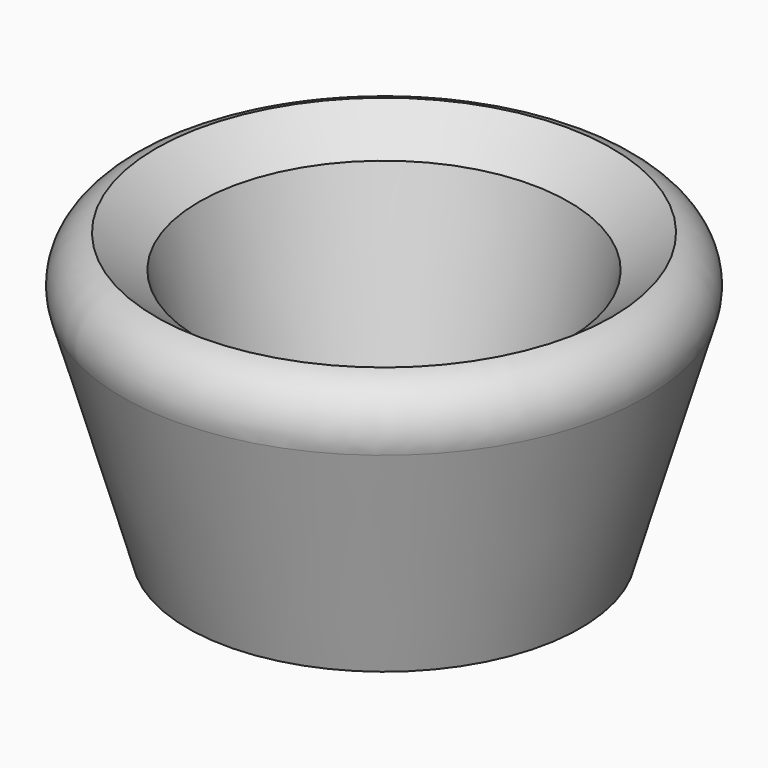
from build123d import *

# Parameters (mm, degrees)
F2_SIZE = 5


# Not quite as in the source:
# - a fillet or chamfer that OpenCascade refuses, or shapes differently, is made with other operations: its cross-section is extruded or revolved along the edge and cut away or added


with BuildPart() as f1:
    # F0 (on Front) → F1 (revolve)
    with BuildSketch(Plane.XZ):
        Polygon((-28.7600811571, 0), (0, 0), (0, 6.0786292888), (-18.5987912118, 6.0786292888), (-28.3971782774, 41.6431464255), (-40.9173406661, 41.6431464255), align=None)
    revolve(axis=Axis((0, 0, 3.0393146444), (0, 0, -1)))

    # F2
    f2_edges = [f1.edges().sort_by_distance(p)[0] for p in [
        (28.397178, 0, 41.643146),
    ]]
    chamfer(f2_edges, length=F2_SIZE)

    # F3: fillet of radius 7 on 1 edges, made by hand

    # F3_s1 → F3_t2 (revolve, cut)
    with BuildSketch(Plane.XZ):
        with BuildLine():
            ThreePointArc((-33.3971782774, 41.6431464255), (-37.73169857, 38.3254350883), (-38.3660170423, 32.9039118006))
            Line((-38.3660170423, 32.9039118006), (-38.5004071994, 32.8646780693))
            Line((-38.5004071994, 32.8646780693), (-41.0517308232, 41.6039126942))
            Line((-41.0517308232, 41.6039126942), (-40.9173406661, 41.7831464255))
            ThreePointArc((-40.9173406661, 41.7831464255), (-37.1572594717, 41.7831464255), (-33.4321916592, 41.7786973867))
            Line((-33.4321916592, 41.7786973867), (-33.3971782774, 41.6431464255))
        make_face()
    revolve(axis=Axis((0, 0, 41.6431464255), (0, 0, -1)), mode=Mode.SUBTRACT)


solid = f1.part
